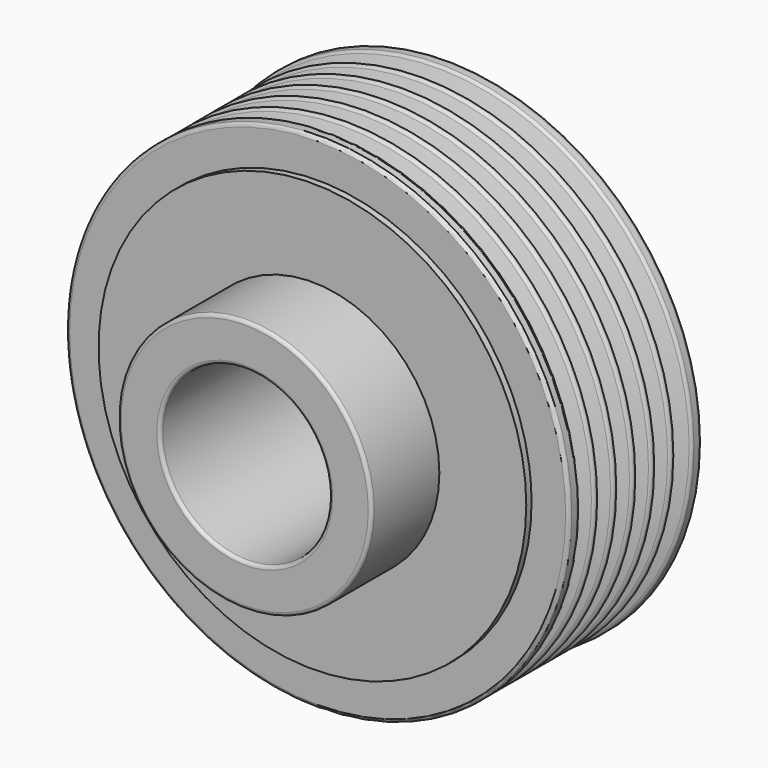
from build123d import *

# Parameters (mm, degrees)
F0_R     = 19.05
F0_R_2   = 12.7
F3_DEPTH = 38.1
F0_R_3   = 32.0923043069
F4_DEPTH = 25.4


# Not quite as in the source:
# - a fillet or chamfer that OpenCascade refuses, or shapes differently, is made with other operations: its cross-section is extruded or revolved along the edge and cut away or added


with BuildPart() as f2:
    # F2: sweep along a path in F0
    with BuildLine(Plane.XZ) as f2_path:
        CenterArc((0, 0), 38.1, 0, 360)
    # F1 (on Right) → F2 (sweep)
    with BuildSketch(Plane.YZ):
        with BuildLine():
            Line((-24.4126301259, 29.4930711389), (0, 29.4930711389))
            Line((0, 29.4930711389), (0, 38.1))
            Line((0, 38.1), (-1.5159870583, 38.1))
            ThreePointArc((-1.5159870583, 38.1), (-1.7771493825, 37.9956074959), (-1.942746962, 37.7682729492))
            Line((-1.942746962, 37.7682729492), (-3.0957230848, 34.6004970869))
            ThreePointArc((-3.0957230848, 34.6004970869), (-3.313880751, 34.4342007842), (-3.5559765663, 34.563184674))
            ThreePointArc((-3.5559765663, 34.563184674), (-3.5652403449, 34.5813935625), (-3.5730107524, 34.6002880585))
            Line((-3.5730107524, 34.6002880585), (-4.6052238569, 37.4285598497))
            ThreePointArc((-4.6052238569, 37.4285598497), (-5.0828802983, 37.7623953652), (-5.5599511934, 37.4277236028))
            Line((-5.5599511934, 37.4277236028), (-6.6258222527, 34.4912666992))
            ThreePointArc((-6.6258222527, 34.4912666992), (-6.8643577003, 34.323930818), (-7.103185921, 34.4908485758))
            Line((-7.103185921, 34.4908485758), (-8.1689408402, 37.4110251954))
            ThreePointArc((-8.1689408402, 37.4110251954), (-8.6463748028, 37.7448608571), (-9.1235161753, 37.4106071386))
            Line((-9.1235161753, 37.4106071386), (-10.1843888499, 34.4958834202))
            ThreePointArc((-10.1843888499, 34.4958834202), (-10.4230707756, 34.3287565366), (-10.6617527013, 34.4958834202))
            Line((-10.6617527013, 34.4958834202), (-11.722464422, 37.4101649213))
            ThreePointArc((-11.722464422, 37.4101649213), (-12.1998282733, 37.7444186885), (-12.6771921247, 37.4101649213))
            Line((-12.6771921247, 37.4101649213), (-13.7403888499, 34.4890559262))
            ThreePointArc((-13.7403888499, 34.4890559262), (-13.9790707756, 34.3219290426), (-14.2177527013, 34.4890559262))
            Line((-14.2177527013, 34.4890559262), (-15.278464422, 37.4033374273))
            ThreePointArc((-15.278464422, 37.4033374273), (-15.7558282733, 37.7375911945), (-16.2331921247, 37.4033374273))
            Line((-16.2331921247, 37.4033374273), (-17.3016348202, 34.4678152474))
            ThreePointArc((-17.3016348202, 34.4678152474), (-17.5403167459, 34.3006883638), (-17.7789986716, 34.4678152474))
            Line((-17.7789986716, 34.4678152474), (-18.8421953968, 37.3889242425))
            ThreePointArc((-18.8421953968, 37.3889242425), (-19.3193367693, 37.723177961), (-19.7967707319, 37.3893422992))
            Line((-19.7967707319, 37.3893422992), (-20.8601960086, 34.4755489182))
            ThreePointArc((-20.8601960086, 34.4755489182), (-21.0989129899, 34.3086310873), (-21.3374836761, 34.4757579466))
            Line((-21.3374836761, 34.4757579466), (-22.3981953968, 37.3900394477))
            ThreePointArc((-22.3981953968, 37.3900394477), (-22.5841824185, 37.6324224534), (-22.8755592482, 37.7242932149))
            Line((-22.8755592482, 37.7242932149), (-24.4126301259, 37.7242932149))
            Line((-24.4126301259, 37.7242932149), (-24.4126301259, 34.4785183216))
            Line((-24.4126301259, 34.4785183216), (-24.4126301259, 29.4930711389))
        make_face()
    sweep(path=f2_path.line)



with BuildPart() as f3:
    # F0 (on Front) → F3 (new body)
    with BuildSketch(Plane.XZ):
        Circle(F0_R)
        Circle(F0_R_2, mode=Mode.SUBTRACT)
    extrude(amount=F3_DEPTH)


with BuildPart() as f2_1:
    add(f2.part)

    add(f3.part)  # F4 merges F3
    # F0 (on Front) → F4 (join)
    with BuildSketch(Plane.XZ):
        Circle(F0_R_3)
        Circle(F0_R, mode=Mode.SUBTRACT)
    extrude(amount=F4_DEPTH)

    # F5: fillet of radius 0.508 on 9 edges, made by hand

    # F5_s1 → F5_t2 (revolve, cut)
    with BuildSketch(Plane.XY):
        with BuildLine():
            ThreePointArc((37.592, 0), (37.9512102448, -0.1487897552), (38.1, -0.508))
            Line((38.1, -0.508), (38.1, 0))
            Line((38.1, 0), (37.592, 0))
        make_face()
    revolve(axis=Axis((0, 0, 0), (0, -1, 0)), mode=Mode.SUBTRACT)

    # F5_s3 → F5_t4 (revolve, cut)
    with BuildSketch(Plane.XY):
        with BuildLine():
            ThreePointArc((38.1, -1.4663027602), (38.0081292385, -1.7576795899), (37.7657462328, -1.9436666116))
            Line((37.7657462328, -1.9436666116), (37.7831208561, -1.9914029967))
            ThreePointArc((37.7831208561, -1.9914029967), (37.7856475724, -1.9904833471), (38.1505473284, -1.521047453))
            Line((38.1505473284, -1.521047453), (38.1508, -1.5159870583))
            Line((38.1508, -1.5159870583), (38.1508, -1.4663027602))
            Line((38.1508, -1.4663027602), (38.1, -1.4663027602))
        make_face()
    revolve(axis=Axis((0, -1.5159870583, 0), (0, -1, 0)), mode=Mode.SUBTRACT)

    # F5_s5 → F5_t6 (revolve, cut)
    with BuildSketch(Plane.XY):
        with BuildLine():
            ThreePointArc((37.2162932149, -24.4126301259), (37.5755034597, -24.2638403707), (37.7242932149, -23.9046301259))
            Line((37.7242932149, -23.9046301259), (37.7242932149, -24.4126301259))
            Line((37.7242932149, -24.4126301259), (37.2162932149, -24.4126301259))
        make_face()
    revolve(axis=Axis((0, -24.4126301259, 0), (0, -1, 0)), mode=Mode.SUBTRACT)

    # F5_s7 → F5_t8 (revolve, cut)
    with BuildSketch(Plane.XY):
        with BuildLine():
            ThreePointArc((19.05, -37.592), (18.9012102448, -37.9512102448), (18.542, -38.1))
            Line((18.542, -38.1), (19.05, -38.1))
            Line((19.05, -38.1), (19.05, -37.592))
        make_face()
    revolve(axis=Axis((0, -38.1, 0), (0, -1, 0)), mode=Mode.SUBTRACT)

    # F5_s9 → F5_t10 (revolve, cut)
    with BuildSketch(Plane.XY):
        with BuildLine():
            ThreePointArc((13.208, -38.1), (12.8487897552, -37.9512102448), (12.7, -37.592))
            Line((12.7, -37.592), (12.7, -38.1))
            Line((12.7, -38.1), (13.208, -38.1))
        make_face()
    revolve(axis=Axis((0, -38.1, 0), (0, -1, 0)), mode=Mode.SUBTRACT)

    # F5_s11 → F5_t12 (revolve, cut)
    with BuildSketch(Plane.XY):
        with BuildLine():
            ThreePointArc((12.7, -0.508), (12.8487897552, -0.1487897552), (13.208, 0))
            Line((13.208, 0), (12.7, 0))
            Line((12.7, 0), (12.7, -0.508))
        make_face()
    revolve(axis=Axis((0, 0, 0), (0, -1, 0)), mode=Mode.SUBTRACT)


solid = f2_1.part
